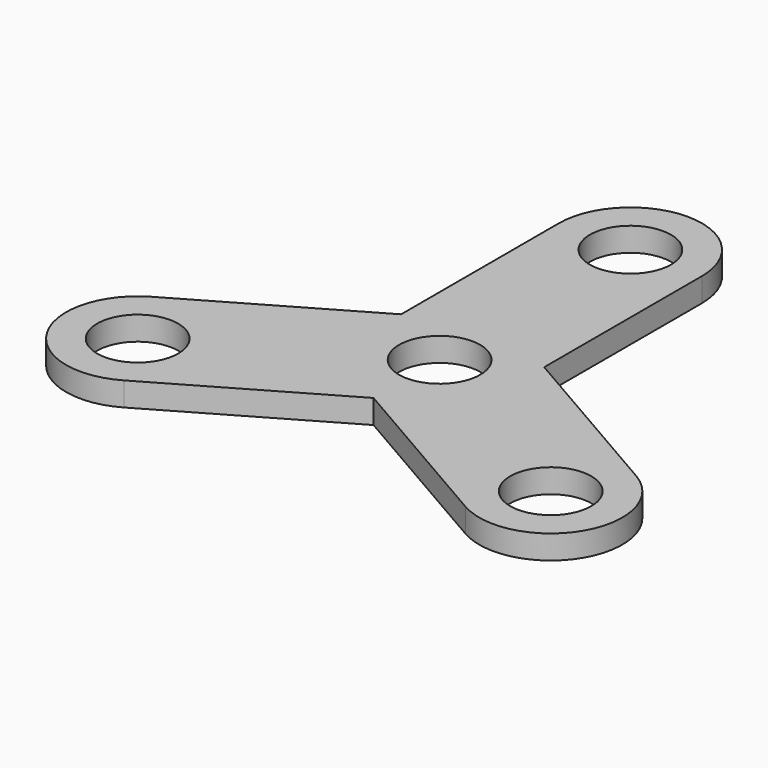
from build123d import *

# Parameters (mm, degrees)
F0_R            = 10.795
F1_DEPTH        = 6.35
F1_COPIES_COUNT = 3


# Not quite as in the source:
# - a pattern or mirror of a feature is missing from the dataset's text; its kind, count and spacing are read off the source's solid


with BuildPart() as f1:
    # F0 (on Top) → F1 (new body)
    with BuildSketch(Plane.XY):
        with BuildLine():
            Line((-19.05, 63.5), (-19.05, 0))
            ThreePointArc((-19.05, 0), (0, -19.05), (19.05, 0))
            Line((19.05, 0), (19.05, 63.5))
            ThreePointArc((19.05, 63.5), (0, 82.55), (-19.05, 63.5))
        make_face()
        Circle(F0_R, mode=Mode.SUBTRACT)
        with Locations((0, 63.5)):
            Circle(F0_R, mode=Mode.SUBTRACT)
    extrude(amount=F1_DEPTH)

    # F1_copies: F1 ×3 about axis
    f1_copies_axis = Axis((0, 0, 0), (0, 0, 1))


with BuildPart() as f1_1:
    add(f1.part)
    for i in range(1, F1_COPIES_COUNT):
        add(f1.part.rotate(f1_copies_axis, i * 360 / F1_COPIES_COUNT))


solid = f1_1.part
